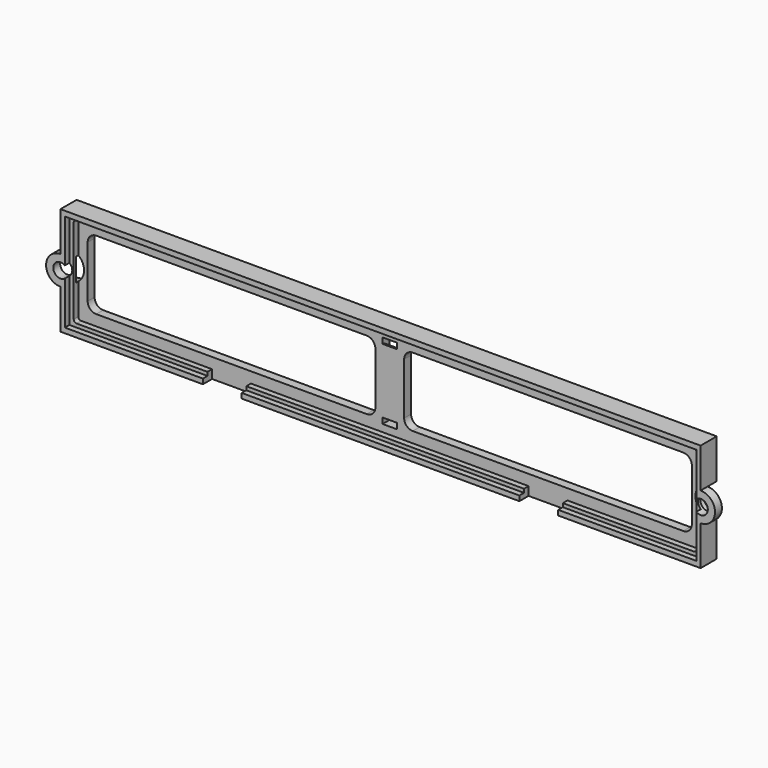
from build123d import *

# Parameters (mm, degrees)
F0_W         = 5
F0_H         = 2
F1_DEPTH     = 3
F2_R         = 2
F3_DEPTH     = 4
F4_W         = 219.5
F4_H         = 34
F4_W_2       = 214.53166008
F4_H_2       = 28.9933998138
F5_DEPTH     = 2
F6_R         = 2.5
F7_DEPTH     = 7.001
F8_R         = 5
F9_DEPTH     = 4
F10_W        = 13.5
F10_H        = 4
F11_DEPTH    = 25
F12_T1_DEPTH = 5


# Not quite as in the source:
# - a fillet or chamfer that OpenCascade refuses, or shapes differently, is made with other operations: its cross-section is extruded or revolved along the edge and cut away or added
# - a feature names something its author has since deleted; it is built from what else it names


with BuildPart() as f1:
    # F0 (on Front) → F1 (new body)
    with BuildSketch(Plane.XZ):
        Polygon((111.25, 5), (111.25, 18.75), (-111.25, 18.75), (-111.25, 5), (-111.25, -5), (-111.25, -18.75), (111.25, -18.75), (111.25, -5), align=None)
        with Locations((0, -12.25)):
            Rectangle(F0_W, F0_H, mode=Mode.SUBTRACT)
        with BuildLine():
            Line((-102, 12), (-8, 12))
            ThreePointArc((-8, 12), (-5.8786796564, 11.1213203436), (-5, 9))
            Line((-5, 9), (-5, -9))
            ThreePointArc((-5, -9), (-5.8786796564, -11.1213203436), (-8, -12))
            Line((-8, -12), (-102, -12))
            ThreePointArc((-102, -12), (-104.1213203436, -11.1213203436), (-105, -9))
            Line((-105, -9), (-105, 9))
            ThreePointArc((-105, 9), (-104.1213203436, 11.1213203436), (-102, 12))
        make_face(mode=Mode.SUBTRACT)
        with BuildLine():
            Line((8, 12), (102, 12))
            ThreePointArc((102, 12), (104.1213203436, 11.1213203436), (105, 9))
            Line((105, 9), (105, -9))
            ThreePointArc((105, -9), (104.1213203436, -11.1213203436), (102, -12))
            Line((102, -12), (8, -12))
            ThreePointArc((8, -12), (5.8786796564, -11.1213203436), (5, -9))
            Line((5, -9), (5, 9))
            ThreePointArc((5, 9), (5.8786796564, 11.1213203436), (8, 12))
        make_face(mode=Mode.SUBTRACT)
        with Locations((0, 12.25)):
            Rectangle(F0_W, F0_H, mode=Mode.SUBTRACT)
        with BuildLine():
            ThreePointArc((111.25, -5), (116.25, 0), (111.25, 5))
            Line((111.25, 5), (111.25, -5))
        make_face()
        with BuildLine():
            Line((-111.25, -5), (-111.25, 5))
            ThreePointArc((-111.25, 5), (-116.25, 0), (-111.25, -5))
        make_face()
    extrude(amount=F1_DEPTH)

    # F2 (on face) → F3 (join)
    with BuildSketch(Plane.XZ.offset(3)):
        with BuildLine():
            ThreePointArc((111.25, -5), (116.25, 0), (111.25, 5))
            Line((111.25, 5), (111.25, 18.75))
            Line((111.25, 18.75), (-111.25, 18.75))
            Line((-111.25, 18.75), (-111.25, 5))
            ThreePointArc((-111.25, 5), (-116.25, 0), (-111.25, -5))
            Line((-111.25, -5), (-111.25, -18.75))
            Line((-111.25, -18.75), (111.25, -18.75))
            Line((111.25, -18.75), (111.25, -5))
        make_face()
        with Locations((-111.25, 0)):
            Circle(F2_R, mode=Mode.SUBTRACT)
        with BuildLine():
            Line((-107.25, 15.75), (107.25, 15.75))
            ThreePointArc((107.25, 15.75), (107.9571067812, 15.4571067812), (108.25, 14.75))
            Line((108.25, 14.75), (108.25, -14.75))
            ThreePointArc((108.25, -14.75), (107.9571067812, -15.4571067812), (107.25, -15.75))
            Line((107.25, -15.75), (-107.25, -15.75))
            ThreePointArc((-107.25, -15.75), (-107.9571067812, -15.4571067812), (-108.25, -14.75))
            Line((-108.25, -14.75), (-108.25, 14.75))
            ThreePointArc((-108.25, 14.75), (-107.9571067812, 15.4571067812), (-107.25, 15.75))
        make_face(mode=Mode.SUBTRACT)
        with Locations((111.25, 0)):
            Circle(F2_R, mode=Mode.SUBTRACT)
    extrude(amount=F3_DEPTH)

    # F4 (on face) → F5 (cut)
    with BuildSketch(Plane.XZ.offset(7)):
        Rectangle(F4_W, F4_H)
        Rectangle(F4_W_2, F4_H_2, mode=Mode.SUBTRACT)
    extrude(amount=-F5_DEPTH, mode=Mode.SUBTRACT)

    # F6 (on face) → F7 (cut, through all)
    with BuildSketch(Plane.XZ.offset(7)):
        with Locations((-111.25, 0)):
            Circle(F6_R)
        with Locations((111.25, 0)):
            Circle(F6_R)
    extrude(amount=-F7_DEPTH, mode=Mode.SUBTRACT)

    # F8 (on face) → F9 (cut)
    with BuildSketch(Plane(origin=(0, 0, 0), x_dir=(-1, 0, 0), z_dir=(0, 1, 0))):
        with Locations((-111.25, 0)):
            Circle(F8_R)
        with Locations((111.25, 0)):
            Circle(F8_R)
    extrude(amount=-F9_DEPTH, mode=Mode.SUBTRACT)

    # F10 (on face) → F11 (cut)
    with BuildSketch(Plane(origin=(0, 0, -18.75), x_dir=(1, 0, 0), z_dir=(0, 0, -1))):
        with Locations((-55, 5)):
            Rectangle(F10_W, F10_H)
        with Locations((55, 5)):
            Rectangle(F10_W, F10_H)
    extrude(amount=-F11_DEPTH, mode=Mode.SUBTRACT)

    # F12: fillet of radius 3.5 on 2 edges, made by hand

    # F12_s2 → F12_t1 (cut)
    with BuildSketch(Plane.YZ.offset(-2.5)):
        with BuildLine():
            ThreePointArc((0, 7.7858983849), (-0.8542486889, 10.0771862323), (-3, 11.25))
            Line((-3, 11.25), (0, 11.25))
            Line((0, 11.25), (0, 7.7858983849))
        make_face()
        with BuildLine():
            ThreePointArc((0, -7.7858983849), (-0.8542486889, -10.0771862323), (-3, -11.25))
            Line((-3, -11.25), (0, -11.25))
            Line((0, -11.25), (0, -7.7858983849))
        make_face()
    extrude(amount=F12_T1_DEPTH, mode=Mode.SUBTRACT)


solid = f1.part
